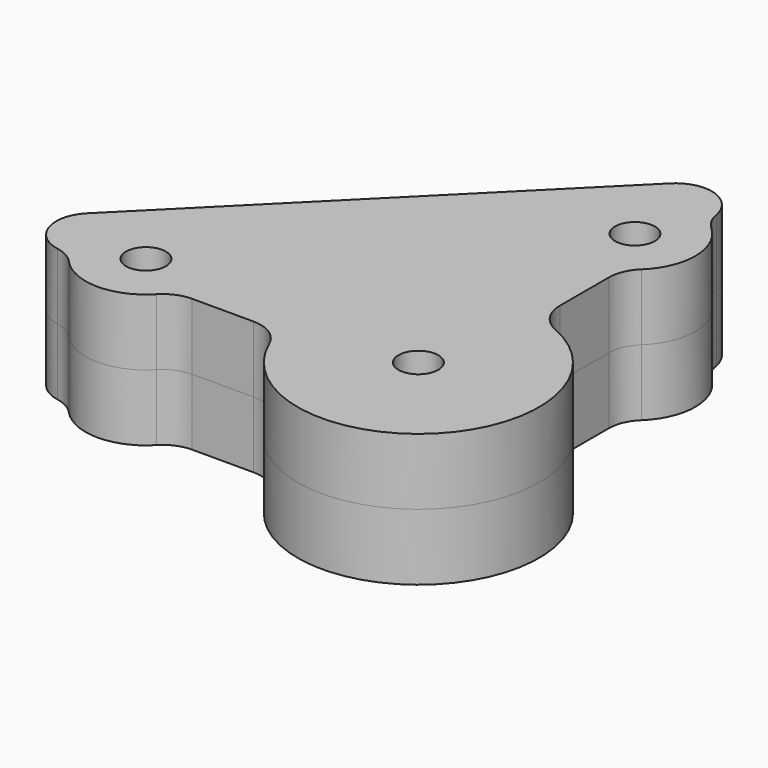
from build123d import *

# Parameters (mm, degrees)
F1_DEPTH = 3
F0_R     = 1.65
F2_DEPTH = 5.5
F3_R     = 3
F4_R     = 3
F5_R     = 1


# Not quite as in the source:
# - a feature names something its author has since deleted; it is built from what else it names


with BuildPart() as f1:
    # F0 (on Top) → F1 (new body)
    with BuildSketch(Plane.XY):
        with BuildLine():
            ThreePointArc((-9.5916630466, 2.8284271247), (-7.0710678119, 7.0710678119), (-2.8284271247, 9.5916630466))
            Line((-2.8284271247, 9.5916630466), (-2.8284271247, 22.8284271247))
            Line((-2.8284271247, 22.8284271247), (-22.8284271247, 2.8284271247))
            Line((-22.8284271247, 2.8284271247), (-9.5916630466, 2.8284271247))
        make_face()
        with BuildLine():
            Line((-2.8284271247, 3.8284271247), (-2.8284271247, 9.5916630466))
            ThreePointArc((-2.8284271247, 9.5916630466), (-7.0710678119, 7.0710678119), (-9.5916630466, 2.8284271247))
            Line((-9.5916630466, 2.8284271247), (-3.8284271247, 2.8284271247))
            ThreePointArc((-3.8284271247, 2.8284271247), (-3.5355339059, 3.5355339059), (-2.8284271247, 3.8284271247))
        make_face()
        Polygon((-22.8284271247, 2.8284271247), (-2.8284271247, 22.8284271247), (-2.8284271247, 29.8994949366), (-29.8994949366, 2.8284271247), align=None)
        with BuildLine():
            ThreePointArc((-1.8284271247, 2.8284271247), (-2.1213203436, 3.5355339059), (-2.8284271247, 3.8284271247))
            Line((-2.8284271247, 3.8284271247), (-2.8284271247, 2.8284271247))
            Line((-2.8284271247, 2.8284271247), (-3.8284271247, 2.8284271247))
            ThreePointArc((-3.8284271247, 2.8284271247), (-2.8284271247, 1.8284271247), (-1.8284271247, 2.8284271247))
        make_face()
        with BuildLine():
            Line((-2.8284271247, 2.8284271247), (-2.8284271247, 3.8284271247))
            ThreePointArc((-2.8284271247, 3.8284271247), (-3.5355339059, 3.5355339059), (-3.8284271247, 2.8284271247))
            Line((-3.8284271247, 2.8284271247), (-2.8284271247, 2.8284271247))
        make_face()
    extrude(amount=F1_DEPTH)

    # F0 (on Top) → F2 (join)
    with BuildSketch(Plane.XY):
        with BuildLine():
            ThreePointArc((-9.7613662593, -2.1715728753), (1.0923226189, -9.9401625387), (10, 0))
            ThreePointArc((10, 0), (7.8011450683, 6.2563676062), (2.1715728753, 9.7613662593))
            ThreePointArc((2.1715728753, 9.7613662593), (-0.3392111015, 9.9942451355), (-2.8284271247, 9.5916630466))
            Line((-2.8284271247, 9.5916630466), (-2.8284271247, 3.8284271247))
            ThreePointArc((-2.8284271247, 3.8284271247), (-2.1213203436, 3.5355339059), (-1.8284271247, 2.8284271247))
            ThreePointArc((-1.8284271247, 2.8284271247), (-2.8284271247, 1.8284271247), (-3.8284271247, 2.8284271247))
            Line((-3.8284271247, 2.8284271247), (-9.5916630466, 2.8284271247))
            ThreePointArc((-9.5916630466, 2.8284271247), (-9.9942451355, 0.3392111015), (-9.7613662593, -2.1715728753))
        make_face()
        Circle(F0_R, mode=Mode.SUBTRACT)
        with BuildLine():
            ThreePointArc((-2.8284271247, 9.5916630466), (-0.3392111015, 9.9942451355), (2.1715728753, 9.7613662593))
            Line((2.1715728753, 9.7613662593), (2.1715728753, 18.4983001058))
            Line((2.1715728753, 18.4983001058), (2.1715728753, 27.1585541437))
            Line((2.1715728753, 27.1585541437), (2.1715728753, 34.8994949366))
            Line((2.1715728753, 34.8994949366), (-2.8284271247, 29.8994949366))
            Line((-2.8284271247, 29.8994949366), (-2.8284271247, 22.8284271247))
            Line((-2.8284271247, 22.8284271247), (-2.8284271247, 9.5916630466))
        make_face()
        with Locations((-0.3284271247, 22.8284271247)):
            Circle(F0_R, mode=Mode.SUBTRACT)
        with BuildLine():
            Line((-18.4983001058, -2.1715728753), (-9.7613662593, -2.1715728753))
            ThreePointArc((-9.7613662593, -2.1715728753), (-9.9942451355, 0.3392111015), (-9.5916630466, 2.8284271247))
            Line((-9.5916630466, 2.8284271247), (-22.8284271247, 2.8284271247))
            Line((-22.8284271247, 2.8284271247), (-29.8994949366, 2.8284271247))
            Line((-29.8994949366, 2.8284271247), (-34.8994949366, -2.1715728753))
            Line((-34.8994949366, -2.1715728753), (-27.1585541437, -2.1715728753))
            Line((-27.1585541437, -2.1715728753), (-18.4983001058, -2.1715728753))
        make_face()
        with Locations((-22.8284271247, 0.3284271247)):
            Circle(F0_R, mode=Mode.SUBTRACT)
        with BuildLine():
            ThreePointArc((-27.1585541437, -2.1715728753), (-22.8284271247, -4.6715728753), (-18.4983001058, -2.1715728753))
            Line((-18.4983001058, -2.1715728753), (-27.1585541437, -2.1715728753))
        make_face()
        with BuildLine():
            Line((2.1715728753, 27.1585541437), (2.1715728753, 18.4983001058))
            ThreePointArc((2.1715728753, 18.4983001058), (4.6715728753, 22.8284271247), (2.1715728753, 27.1585541437))
        make_face()
    extrude(amount=F2_DEPTH)

    # F3
    f3_edges = [f1.edges().sort_by_distance(p)[0] for p in [
        (2.171573, 34.899495, 2.75),
        (-34.899495, -2.171573, 2.75),
    ]]
    fillet(f3_edges, radius=F3_R)

    # F4
    f4_edges = [f1.edges().sort_by_distance(p)[0] for p in [
        (-9.761366, -2.171573, 2.75),
        (2.171573, 9.761366, 2.75),
        (-27.158554, -2.171573, 2.75),
        (2.171573, 27.158554, 2.75),
        (-18.4983, -2.171573, 2.75),
        (2.171573, 18.4983, 2.75),
    ]]
    fillet(f4_edges, radius=F4_R)

    # F5
    f5_edges = [f1.edges().sort_by_distance(p)[0] for p in [
        (-2.828427, 29.892922, 4.25),
        (-29.892922, 2.828427, 4.25),
        (-2.828427, 3.828427, 4.25),
        (-3.828427, 2.828427, 4.25),
    ]]
    fillet(f5_edges, radius=F5_R)


with BuildPart() as f6_1:
    # F6: instance of F1
    add(f1.part.mirror(Plane(origin=(-4.0944807871, 4.0944807939, 5.5), x_dir=(1, 0, 0), z_dir=(0, 0, 1))))


solid = Compound([f1.part, f6_1.part])
